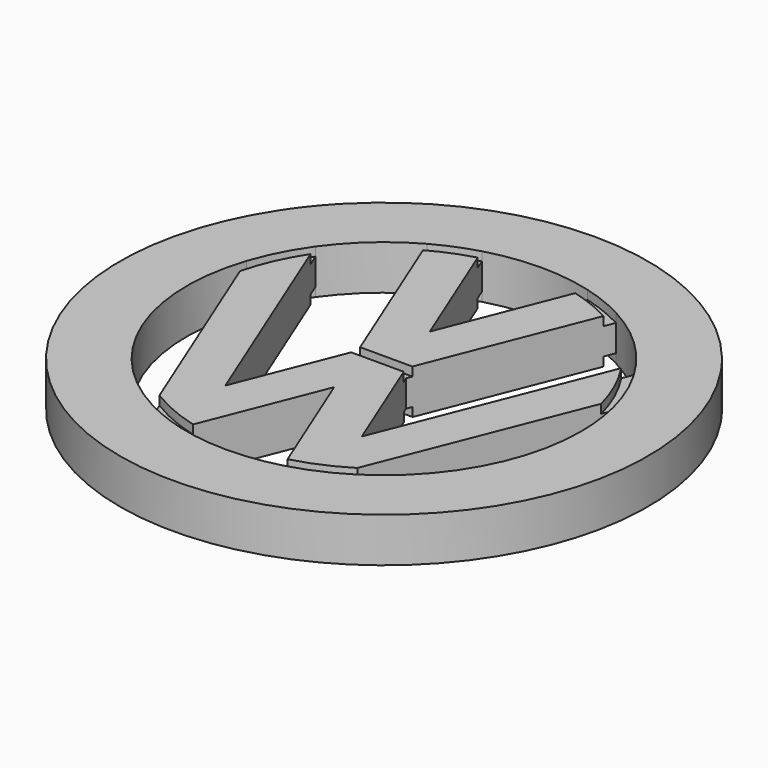
from build123d import *

# Parameters (mm, degrees)
F1_DEPTH  = 20
F3_DEPTH  = 20
F2_R      = 88.5
F2_R_2    = 83.5
F4_DEPTH  = 4
F6_DEPTH  = 4
F8_DEPTH  = 4
F10_DEPTH = 4


with BuildPart() as f1:
    # F0 (on Top) → F1 (new body)
    with BuildSketch(Plane.XY):
        with BuildLine():
            ThreePointArc((-99.0167204009, 65.0994553054), (-33.976231637, -113.5247359995), (118.5, 0))
            ThreePointArc((118.5, 0), (113.427568701, 34.2992224195), (98.6445289691, 65.6620659473))
            Line((98.6445289691, 65.6620659473), (83.8359894773, 28.3509588615))
            ThreePointArc((83.8359894773, 28.3509588615), (87.3262133289, 14.3660177374), (88.5, 0))
            ThreePointArc((88.5, 0), (75.9227513097, -45.4751122436), (41.7658568686, -78.0247601729))
            ThreePointArc((41.7658568686, -78.0247601729), (37.4975464632, -80.1634830159), (33.1201145514, -82.0689223282))
            ThreePointArc((33.1201145514, -82.0689223282), (28.1992209584, -83.8871500132), (23.1792402745, -85.4106130425))
            ThreePointArc((23.1792402745, -85.4106130425), (0.1291202837, -88.4999058076), (-22.9299160381, -85.4778857395))
            ThreePointArc((-22.9299160381, -85.4778857395), (-27.7305413867, -84.0432452634), (-32.4422838504, -82.3392264876))
            ThreePointArc((-32.4422838504, -82.3392264876), (-37.0493645428, -80.3716031131), (-41.5377286395, -78.1464464929))
            ThreePointArc((-41.5377286395, -78.1464464929), (-82.1619405668, -32.888683803), (-83.9871522499, 27.8999687625))
            Line((-83.9871522499, 27.8999687625), (-99.0167204009, 65.0994553054))
        make_face()
        with BuildLine():
            Line((83.8359894773, 28.3509588615), (98.6445289691, 65.6620659473))
            ThreePointArc((98.6445289691, 65.6620659473), (95.2609020622, 70.4812779275), (91.6420527878, 75.1264544673))
            Line((91.6420527878, 75.1264544673), (78.2404891828, 41.3603173639))
            ThreePointArc((78.2404891828, 41.3603173639), (81.2988750591, 34.9677410499), (83.8359894773, 28.3509588615))
        make_face()
        with BuildLine():
            ThreePointArc((-91.7323358048, 75.0161887049), (-95.5033298433, 70.1524339481), (-99.0167204009, 65.0994553054))
            Line((-99.0167204009, 65.0994553054), (-83.9871522499, 27.8999687625))
            ThreePointArc((-83.9871522499, 27.8999687625), (-81.3673031633, 34.8082170749), (-78.1803580333, 41.4738666848))
            Line((-78.1803580333, 41.4738666848), (-91.7323358048, 75.0161887049))
        make_face()
        with BuildLine():
            Line((78.2404891828, 41.3603173639), (91.6420527878, 75.1264544673))
            ThreePointArc((91.6420527878, 75.1264544673), (88.0042632721, 79.3567870187), (84.1713836102, 83.4111993748))
            Line((84.1713836102, 83.4111993748), (71.6717000696, 51.9174094994))
            ThreePointArc((71.6717000696, 51.9174094994), (75.141727224, 46.7543669597), (78.2404891828, 41.3603173639))
        make_face()
        with BuildLine():
            ThreePointArc((-84.6487172303, 82.9267427991), (-88.279177522, 79.0508495593), (-91.7323358048, 75.0161887049))
            Line((-91.7323358048, 75.0161887049), (-78.1803580333, 41.4738666848))
            ThreePointArc((-78.1803580333, 41.4738666848), (-75.2374774209, 46.6001286623), (-71.9589677924, 51.5185107923))
            Line((-71.9589677924, 51.5185107923), (-84.6487172303, 82.9267427991))
        make_face()
        with BuildLine():
            Line((71.6717000696, 51.9174094994), (84.1713836102, 83.4111993748))
            ThreePointArc((84.1713836102, 83.4111993748), (-0.34005351, 118.4995120817), (-84.6487172303, 82.9267427991))
            Line((-84.6487172303, 82.9267427991), (-71.9589677924, 51.5185107923))
            ThreePointArc((-71.9589677924, 51.5185107923), (-58.7666735297, 66.1719584285), (-42.657447205, 77.5409066104))
            ThreePointArc((-42.657447205, 77.5409066104), (-37.9880889567, 79.9321906207), (-33.1852472612, 82.0426070052))
            ThreePointArc((-33.1852472612, 82.0426070052), (-28.7127568961, 83.7127683894), (-24.1567096164, 85.1393174774))
            ThreePointArc((-24.1567096164, 85.1393174774), (-0.5199906824, 88.4984723579), (23.1545696711, 85.4173044725))
            ThreePointArc((23.1545696711, 85.4173044725), (27.9506996195, 83.9702827837), (32.6572676565, 82.2541966663))
            ThreePointArc((32.6572676565, 82.2541966663), (37.2598684434, 80.274231255), (41.7430426186, 78.0369681173))
            ThreePointArc((41.7430426186, 78.0369681173), (58.1917846466, 66.6780788538), (71.6717000696, 51.9174094994))
        make_face()
    extrude(amount=F1_DEPTH)

    # F0 (on Top) → F3 (join)
    with BuildSketch(Plane.XY):
        Polygon((-5.3900272877, 13.2470234608), (-10.9754492604, -0.8747899922), (-5.5413465001, -14.3246662942), (0.0440754726, -0.2028528412), align=None)
        Polygon((-5.5413465001, -14.3246662942), (-0.1072437399, -27.7745425962), (5.4781782329, -13.6527291432), (0.0440754726, -0.2028528412), align=None)
        Polygon((5.4781782329, -13.6527291432), (10.5633239718, -0.7957812068), (5.1292212115, 12.6540950952), (0.0440754726, -0.2028528412), align=None)
        Polygon((0.0440754726, -0.2028528412), (5.1292212115, 12.6540950952), (-0.3048815487, 26.1039713972), (-5.3900272877, 13.2470234608), align=None)
        Polygon((-10.9754492604, -0.8747899922), (-30.6712140088, -50.6722658047), (-25.2371112485, -64.1221421067), (-5.5413465001, -14.3246662942), align=None)
        with BuildLine():
            Line((-25.2371112485, -64.1221421067), (-32.4422838504, -82.3392264876))
            ThreePointArc((-32.4422838504, -82.3392264876), (-27.7305413867, -84.0432452634), (-22.9299160381, -85.4778857395))
            Line((-22.9299160381, -85.4778857395), (-0.1072437399, -27.7745425962))
            Line((-0.1072437399, -27.7745425962), (-5.5413465001, -14.3246662942))
            Line((-5.5413465001, -14.3246662942), (-25.2371112485, -64.1221421067))
        make_face()
        with BuildLine():
            Line((-41.3417817205, -77.6510271941), (-41.5377286395, -78.1464464929))
            ThreePointArc((-41.5377286395, -78.1464464929), (-37.0493645428, -80.3716031131), (-32.4422838504, -82.3392264876))
            Line((-32.4422838504, -82.3392264876), (-25.2371112485, -64.1221421067))
            Line((-25.2371112485, -64.1221421067), (-30.6712140088, -50.6722658047))
            Line((-30.6712140088, -50.6722658047), (-35.7563597477, -63.5292137411))
            Line((-35.7563597477, -63.5292137411), (-41.3417817205, -77.6510271941))
        make_face()
        with BuildLine():
            ThreePointArc((-71.9589677924, 51.5185107923), (-75.2374774209, 46.6001286623), (-78.1803580333, 41.4738666848))
            Line((-78.1803580333, 41.4738666848), (-35.7563597477, -63.5292137411))
            Line((-35.7563597477, -63.5292137411), (-30.6712140088, -50.6722658047))
            Line((-30.6712140088, -50.6722658047), (-71.9589677924, 51.5185107923))
        make_face()
        with BuildLine():
            ThreePointArc((-78.1803580333, 41.4738666848), (-81.3673031633, 34.8082170749), (-83.9871522499, 27.8999687625))
            Line((-83.9871522499, 27.8999687625), (-41.3417817205, -77.6510271941))
            Line((-41.3417817205, -77.6510271941), (-35.7563597477, -63.5292137411))
            Line((-35.7563597477, -63.5292137411), (-78.1803580333, 41.4738666848))
        make_face()
        with BuildLine():
            Line((5.1292212115, 12.6540950952), (32.6572676565, 82.2541966663))
            ThreePointArc((32.6572676565, 82.2541966663), (27.9506996195, 83.9702827837), (23.1545696711, 85.4173044725))
            Line((23.1545696711, 85.4173044725), (-0.3048815487, 26.1039713972))
            Line((-0.3048815487, 26.1039713972), (5.1292212115, 12.6540950952))
        make_face()
        with BuildLine():
            Line((10.5633239718, -0.7957812068), (41.7430426186, 78.0369681173))
            ThreePointArc((41.7430426186, 78.0369681173), (37.2598684434, 80.274231255), (32.6572676565, 82.2541966663))
            Line((32.6572676565, 82.2541966663), (5.1292212115, 12.6540950952))
            Line((5.1292212115, 12.6540950952), (10.5633239718, -0.7957812068))
        make_face()
        with BuildLine():
            ThreePointArc((-33.1852472612, 82.0426070052), (-37.9880889567, 79.9321906207), (-42.657447205, 77.5409066104))
            Line((-42.657447205, 77.5409066104), (-10.9754492604, -0.8747899922))
            Line((-10.9754492604, -0.8747899922), (-5.3900272877, 13.2470234608))
            Line((-5.3900272877, 13.2470234608), (-33.1852472612, 82.0426070052))
        make_face()
        with BuildLine():
            ThreePointArc((-24.1567096164, 85.1393174774), (-28.7127568961, 83.7127683894), (-33.1852472612, 82.0426070052))
            Line((-33.1852472612, 82.0426070052), (-5.3900272877, 13.2470234608))
            Line((-5.3900272877, 13.2470234608), (-0.3048815487, 26.1039713972))
            Line((-0.3048815487, 26.1039713972), (-24.1567096164, 85.1393174774))
        make_face()
        with BuildLine():
            ThreePointArc((23.1792402745, -85.4106130425), (28.1992209584, -83.8871500132), (33.1201145514, -82.0689223282))
            Line((33.1201145514, -82.0689223282), (25.7416192077, -63.806505505))
            Line((25.7416192077, -63.806505505), (5.4781782329, -13.6527291432))
            Line((5.4781782329, -13.6527291432), (-0.1072437399, -27.7745425962))
            Line((-0.1072437399, -27.7745425962), (23.1792402745, -85.4106130425))
        make_face()
        Polygon((25.7416192077, -63.806505505), (30.8356910223, -50.971650381), (10.5633239718, -0.7957812068), (5.4781782329, -13.6527291432), align=None)
        with BuildLine():
            Line((41.7658568686, -78.0247601729), (41.6903356821, -77.8378386773))
            Line((41.6903356821, -77.8378386773), (36.2630133522, -64.4047445292))
            Line((36.2630133522, -64.4047445292), (30.8356910223, -50.971650381))
            Line((30.8356910223, -50.971650381), (25.7416192077, -63.806505505))
            Line((25.7416192077, -63.806505505), (33.1201145514, -82.0689223282))
            ThreePointArc((33.1201145514, -82.0689223282), (37.4975464632, -80.1634830159), (41.7658568686, -78.0247601729))
        make_face()
        with BuildLine():
            Line((41.6903356821, -77.8378386773), (83.8359894773, 28.3509588615))
            ThreePointArc((83.8359894773, 28.3509588615), (81.2988750591, 34.9677410499), (78.2404891828, 41.3603173639))
            Line((78.2404891828, 41.3603173639), (36.2630133522, -64.4047445292))
            Line((36.2630133522, -64.4047445292), (41.6903356821, -77.8378386773))
        make_face()
        with BuildLine():
            Line((36.2630133522, -64.4047445292), (78.2404891828, 41.3603173639))
            ThreePointArc((78.2404891828, 41.3603173639), (75.141727224, 46.7543669597), (71.6717000696, 51.9174094994))
            Line((71.6717000696, 51.9174094994), (30.8356910223, -50.971650381))
            Line((30.8356910223, -50.971650381), (36.2630133522, -64.4047445292))
        make_face()
    extrude(amount=F3_DEPTH)

    # F2 (on face) → F4 (cut)
    with BuildSketch(Plane.XY.offset(20)):
        Circle(F2_R)
        Circle(F2_R_2, mode=Mode.SUBTRACT)
    extrude(amount=-F4_DEPTH, mode=Mode.SUBTRACT)

    # F5 (on face) → F6 (cut)
    with BuildSketch(Plane(origin=(0, 0, 0), x_dir=(1, 0, 0), z_dir=(0, 0, -1))):
        with BuildLine():
            ThreePointArc((83.8359894773, -28.3509588615), (87.3262133289, -14.3660177374), (88.5, 0))
            ThreePointArc((88.5, 0), (-27.0544021406, 84.2633332168), (-71.9589677924, -51.5185107923))
            ThreePointArc((-71.9589677924, -51.5185107923), (-58.7666735297, -66.1719584285), (-42.657447205, -77.5409066104))
            ThreePointArc((-42.657447205, -77.5409066104), (-33.6224158838, -81.8644193172), (-24.1567096164, -85.1393174774))
            ThreePointArc((-24.1567096164, -85.1393174774), (-0.5199906824, -88.4984723579), (23.1545696711, -85.4173044725))
            ThreePointArc((23.1545696711, -85.4173044725), (32.6579601538, -82.2539217217), (41.7430426186, -78.0369681173))
            ThreePointArc((41.7430426186, -78.0369681173), (58.1917846466, -66.6780788538), (71.6717000696, -51.9174094994))
            ThreePointArc((71.6717000696, -51.9174094994), (78.6416224144, -40.5924281613), (83.8359894773, -28.3509588615))
        make_face()
        with BuildLine():
            ThreePointArc((44.555375213, 70.6191796868), (73.1184786162, 40.3229225734), (83.5, 0))
            ThreePointArc((83.5, 0), (82.836495174, -10.5054779659), (80.8565253343, -20.843999397))
            ThreePointArc((80.8565253343, -20.843999397), (76.2315862582, -34.0733804687), (69.4592219568, -46.3429227084))
            ThreePointArc((69.4592219568, -46.3429227084), (56.3186534083, -61.6478651559), (39.8912046999, -73.3549029554))
            ThreePointArc((39.8912046999, -73.3549029554), (30.8190728646, -77.6043474798), (21.3033189694, -80.7367239915))
            ThreePointArc((21.3033189694, -80.7367239915), (-0.501796062, -83.4984922062), (-22.2721428532, -80.4748510575))
            ThreePointArc((-22.2721428532, -80.4748510575), (-31.7497249631, -77.2282653228), (-40.7702727747, -72.8699859879))
            ThreePointArc((-40.7702727747, -72.8699859879), (-56.8567093495, -61.1519795423), (-69.7131848128, -45.9600028639))
            ThreePointArc((-69.7131848128, -45.9600028639), (-76.4136411743, -33.6631169454), (-80.9647996196, -20.4193835008))
            ThreePointArc((-80.9647996196, -20.4193835008), (-77.4198518563, 31.2796505502), (-44.0567071244, 70.9313510188))
            ThreePointArc((-44.0567071244, 70.9313510188), (-32.938761393, 76.7286647733), (-21.0780781193, 80.7958205775))
            ThreePointArc((-21.0780781193, 80.7958205775), (0.1106131959, 83.4999267348), (21.2920658442, 80.7396924201))
            ThreePointArc((21.2920658442, 80.7396924201), (33.3103222431, 76.5680901685), (44.555375213, 70.6191796868))
        make_face(mode=Mode.SUBTRACT)
    extrude(amount=-F6_DEPTH, mode=Mode.SUBTRACT)

    # F7 (on face) → F8 (cut)
    with BuildSketch(Plane.XY.offset(20)):
        Polygon((11.4983377003, 1.5682459902), (-11.9624998679, 1.5682459902), (-10.9754492604, -0.8747899922), (-11.9867728454, -3.4317540098), (11.6283261148, -3.4317540098), (10.5633239718, -0.7957812068), align=None)
    extrude(amount=-F8_DEPTH, mode=Mode.SUBTRACT)

    # F9 (on face) → F10 (cut)
    with BuildSketch(Plane(origin=(0, 0, 0), x_dir=(1, 0, 0), z_dir=(0, 0, -1))):
        Polygon((11.5868667585, 3.329138502), (-11.9461866336, 3.329138502), (-10.9754492604, 0.8747899922), (-12.0039592243, -1.670861498), (11.5389239122, -1.670861498), (10.5633239718, 0.7957812068), align=None)
    extrude(amount=-F10_DEPTH, mode=Mode.SUBTRACT)


solid = f1.part
